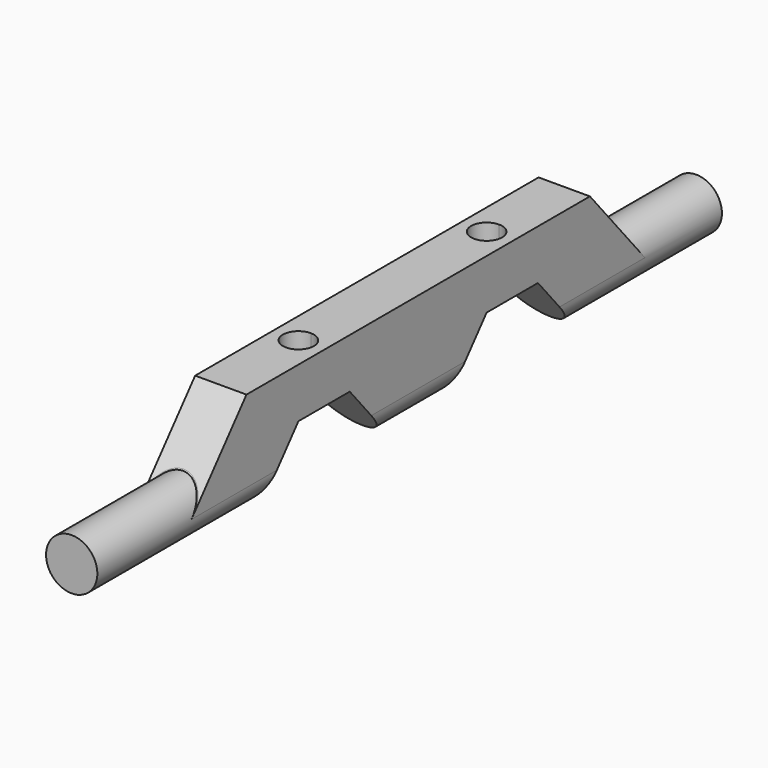
from build123d import *

# Parameters (mm, degrees)
F0_R      = 2.5
F1_DEPTH  = 85
F3_DEPTH  = 2.5
F5_DEPTH  = 25
F8_DEPTH  = 25
F9_DEPTH  = 25
F11_DEPTH = 25
F14_DEPTH = 102
F16_REACH = 96.5783545855
F18_REACH = 97.7333268634
F19_W     = 5
F19_H     = 41.5
F20_DEPTH = 25


with BuildPart() as f1:
    # F0 (on Front) → F1 (new body)
    with BuildSketch(Plane.XZ):
        Circle(F0_R)
    extrude(amount=F1_DEPTH)

    # F2 (on Right) → F3 (join, symmetric)
    with BuildSketch(Plane.YZ):
        Polygon((-69, 0), (-16, 0), (-22.4278760969, 7.6604444312), (-62.5721239031, 7.6604444312), align=None)
    extrude(amount=F3_DEPTH, both=True)

    # F4 (on face) → F5 (cut)
    with BuildSketch(Plane(origin=(-2.5, 0, 0), x_dir=(0, -1, 0), z_dir=(-1, 0, 0))):
        Polygon((56.5, 3), (53.5, 3), (50.5, 3), (44.1691353238, -4.5448307221), (62.8308646762, -4.5448307221), align=None)
        Polygon((40.8308646762, -4.5448307221), (34.5, 3), (31.5, 3), (28.5, 3), (22.1691353238, -4.5448307221), align=None)
    extrude(amount=-F5_DEPTH, mode=Mode.SUBTRACT)

    # F7 (on face) → F8 (cut)
    with BuildSketch(Plane(origin=(-2.5, 0, 0), x_dir=(0, -1, 0), z_dir=(-1, 0, 0))):
        Polygon((19.9172031134, 7.5), (22.2932472338, 7.5), (22.4278760969, 7.6604444312), (62.5721239031, 7.6604444312), (62.7067527662, 7.5), (66.5233954787, 7.5), (66.5233954787, 10.3880958632), (19.9172031134, 10.3880958632), align=None)
    extrude(amount=-F8_DEPTH, mode=Mode.SUBTRACT)

    # F6 (on face) → F9 (cut)
    with BuildSketch(Plane(origin=(0, 0, 3), x_dir=(1, 0, 0), z_dir=(0, 0, -1))):
        with BuildLine():
            ThreePointArc((1.45, 53.5), (1.0253048327, 54.5253048327), (0, 54.95))
            Line((0, 54.95), (0, 52.05))
            ThreePointArc((0, 52.05), (1.0253048327, 52.4746951673), (1.45, 53.5))
        make_face()
        with BuildLine():
            Line((0, 52.05), (0, 54.95))
            ThreePointArc((0, 54.95), (-1.45, 53.5), (0, 52.05))
        make_face()
    extrude(amount=-F9_DEPTH, mode=Mode.SUBTRACT)

    # F10 (on face) → F11 (cut)
    with BuildSketch(Plane(origin=(0, 0, 3), x_dir=(1, 0, 0), z_dir=(0, 0, -1))):
        with BuildLine():
            ThreePointArc((1.45, 31.5), (1.0253048327, 32.5253048327), (0, 32.95))
            Line((0, 32.95), (0, 30.05))
            ThreePointArc((0, 30.05), (1.0253048327, 30.4746951673), (1.45, 31.5))
        make_face()
        with BuildLine():
            Line((0, 30.05), (0, 32.95))
            ThreePointArc((0, 32.95), (-1.45, 31.5), (0, 30.05))
        make_face()
    extrude(amount=-F11_DEPTH, mode=Mode.SUBTRACT)

    # F13 (on face) → F14 (cut)
    with BuildSketch(Plane.XZ.offset(85)):
        with BuildLine():
            ThreePointArc((2.4, 0), (0, -2.4), (-2.4, 0))
            Line((-2.4, 0), (-2.4, 9.7710704431))
            Line((-2.4, 9.7710704431), (-6.1972029507, 9.7710704431))
            Line((-6.1972029507, 9.7710704431), (-6.1972029507, -5.7614380494))
            Line((-6.1972029507, -5.7614380494), (5.5722752586, -5.7614380494))
            Line((5.5722752586, -5.7614380494), (5.5722752586, 8.8547384366))
            Line((5.5722752586, 8.8547384366), (2.4, 9.1607915238))
            Line((2.4, 9.1607915238), (2.4, 0))
        make_face()
    extrude(amount=-F14_DEPTH, mode=Mode.SUBTRACT)

    f16_end = Plane(origin=(0, -64.9529870595, 4.8230422111), x_dir=(0, -0.6427876097, -0.7660444431), z_dir=(0, -0.7660444431, 0.6427876097))
    # F15 (on face) → F16 (cut, up to a plane its end follows)
    with BuildSketch(Plane.XZ.offset(85)):
        with BuildLine():
            ThreePointArc((-2.4, 0), (0, 2.4), (2.4, 0))
            Line((2.4, 0), (4.8319334164, 0))
            Line((4.8319334164, 0), (4.1808704846, 8.0774491653))
            Line((4.1808704846, 8.0774491653), (-2.9383567162, 8.0774491653))
            Line((-2.9383567162, 8.0774491653), (-3.4620375372, 0))
            Line((-3.4620375372, 0), (-2.4, 0))
        make_face()
    f16_long = extrude(amount=-F16_REACH, mode=Mode.PRIVATE)
    add(split(f16_long, bisect_by=f16_end, keep=Keep.TOP, mode=Mode.PRIVATE), mode=Mode.SUBTRACT)

    f18_end = Plane(origin=(0, -20.0470129405, 4.8230422111), x_dir=(0, -0.6427876097, 0.7660444431), z_dir=(0, 0.7660444431, 0.6427876097))
    # F17 (on face) → F18 (cut, up to a plane its end follows)
    with BuildSketch(Plane(origin=(0, 0, 0), x_dir=(-1, 0, 0), z_dir=(0, 1, 0))):
        with BuildLine():
            ThreePointArc((-2.4, 0), (0, 2.4), (2.4, 0))
            Line((2.4, 0), (3.9089121856, 0))
            Line((3.9089121856, 0), (4.3247276917, 8.6870230734))
            Line((4.3247276917, 8.6870230734), (-4.9837511033, 8.3660408854))
            Line((-4.9837511033, 8.3660408854), (-3.4170385916, 0))
            Line((-3.4170385916, 0), (-2.4, 0))
        make_face()
    f18_long = extrude(amount=-F18_REACH, mode=Mode.PRIVATE)
    add(split(f18_long, bisect_by=f18_end, keep=Keep.TOP, mode=Mode.PRIVATE), mode=Mode.SUBTRACT)

    # F19 (on face) → F20 (cut)
    with BuildSketch(Plane.YZ.offset(2.4)):
        Polygon((0, -4.5159468427), (0, -2.4), (0, 2.4), (-7, 2.4), (-7, -4.5159468427), align=None)
        with Locations((-82.5, 0)):
            Rectangle(F19_W, F19_H)
    extrude(amount=-F20_DEPTH, mode=Mode.SUBTRACT)


solid = f1.part
